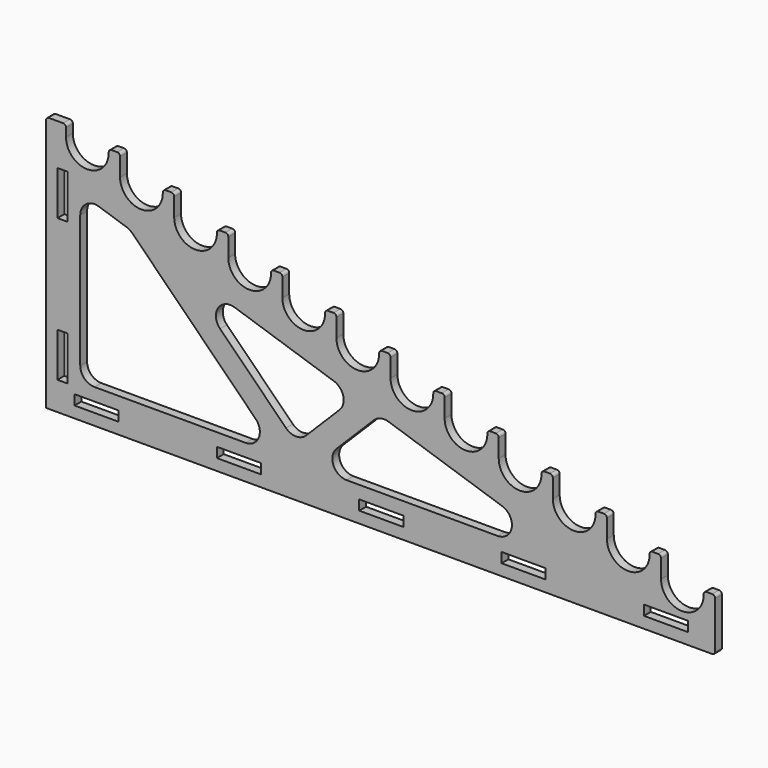
from build123d import *

# Parameters (mm, degrees)
F1_DEPTH = 3
F2_R     = 1
F3_W     = 15.5
F3_H     = 3.5
F3_W_2   = 3.5
F3_H_2   = 15.5
F4_DEPTH = 25


with BuildPart() as f1:
    # F0 (on Front) → F1 (new body)
    with BuildSketch(Plane.XZ):
        with BuildLine():
            Line((0, 90), (0, 0))
            Line((0, 0), (235, 0))
            Line((235, 0), (235, 17.5337082297))
            ThreePointArc((235, 17.5337082297), (234.7071067812, 18.2408150109), (234, 18.5337082297))
            Line((234, 18.5337082297), (232, 18.5337082297))
            ThreePointArc((232, 18.5337082297), (231.2928932188, 18.2408150109), (231, 17.5337082297))
            Line((231, 17.5337082297), (231, 17.3050220176))
            ThreePointArc((231, 17.3050220176), (223.5, 9.8050220176), (216, 17.3050220176))
            Line((216, 17.3050220176), (216, 21.3050220176))
            Line((216, 21.3050220176), (216, 23.7787062281))
            ThreePointArc((216, 23.7787062281), (215.7071067812, 24.4858130093), (215, 24.7787062281))
            Line((215, 24.7787062281), (213, 24.7787062281))
            ThreePointArc((213, 24.7787062281), (212.2928932188, 24.4858130093), (212, 23.7787062281))
            Line((212, 23.7787062281), (212, 23.550020016))
            ThreePointArc((212, 23.550020016), (204.5, 16.050020016), (197, 23.550020016))
            Line((197, 23.550020016), (197, 27.550020016))
            Line((197, 27.550020016), (197, 30.0237042265))
            ThreePointArc((197, 30.0237042265), (196.7071067812, 30.7308110077), (196, 31.0237042265))
            Line((196, 31.0237042265), (194, 31.0237042265))
            ThreePointArc((194, 31.0237042265), (193.2928932188, 30.7308110077), (193, 30.0237042265))
            Line((193, 30.0237042265), (193, 29.7950180144))
            ThreePointArc((193, 29.7950180144), (185.5, 22.2950180144), (178, 29.7950180144))
            Line((178, 29.7950180144), (178, 33.7950180144))
            Line((178, 33.7950180144), (178, 36.2687022249))
            ThreePointArc((178, 36.2687022249), (177.7071067812, 36.9758090061), (177, 37.2687022249))
            Line((177, 37.2687022249), (175, 37.2687022249))
            ThreePointArc((175, 37.2687022249), (174.2928932188, 36.9758090061), (174, 36.2687022249))
            Line((174, 36.2687022249), (174, 36.0400160128))
            ThreePointArc((174, 36.0400160128), (166.5, 28.5400160128), (159, 36.0400160128))
            Line((159, 36.0400160128), (159, 40.0400160128))
            Line((159, 40.0400160128), (159, 42.5137002233))
            ThreePointArc((159, 42.5137002233), (158.7071067812, 43.2208070045), (158, 43.5137002233))
            Line((158, 43.5137002233), (156, 43.5137002233))
            ThreePointArc((156, 43.5137002233), (155.2928932188, 43.2208070045), (155, 42.5137002233))
            Line((155, 42.5137002233), (155, 42.2850140112))
            ThreePointArc((155, 42.2850140112), (147.5, 34.7850140112), (140, 42.2850140112))
            Line((140, 42.2850140112), (140, 46.2850140112))
            Line((140, 46.2850140112), (140, 48.7586982217))
            ThreePointArc((140, 48.7586982217), (139.7071067812, 49.4658050029), (139, 49.7586982217))
            Line((139, 49.7586982217), (137, 49.7586982217))
            ThreePointArc((137, 49.7586982217), (136.2928932188, 49.4658050029), (136, 48.7586982217))
            Line((136, 48.7586982217), (136, 48.5300120096))
            ThreePointArc((136, 48.5300120096), (128.5, 41.0300120096), (121, 48.5300120096))
            Line((121, 48.5300120096), (121, 52.5300120096))
            Line((121, 52.5300120096), (121, 55.0036962201))
            ThreePointArc((121, 55.0036962201), (120.7071067812, 55.7108030013), (120, 56.0036962201))
            Line((120, 56.0036962201), (118, 56.0036962201))
            ThreePointArc((118, 56.0036962201), (117.2928932188, 55.7108030013), (117, 55.0036962201))
            Line((117, 55.0036962201), (117, 54.775010008))
            ThreePointArc((117, 54.775010008), (109.5, 47.275010008), (102, 54.775010008))
            Line((102, 54.775010008), (102, 58.775010008))
            Line((102, 58.775010008), (102, 61.2451730918))
            ThreePointArc((102, 61.2451730918), (101.7058629727, 61.9535214974), (100.9964850724, 62.2451669144))
            Line((100.9964850724, 62.2451669144), (98.9964850724, 62.2381370157))
            ThreePointArc((98.9964850724, 62.2381370157), (98.2916515943, 61.9440061658), (98, 61.2381431931))
            Line((98, 61.2381431931), (98, 61.0200080064))
            ThreePointArc((98, 61.0200080064), (90.5, 53.5200080064), (83, 61.0200080064))
            Line((83, 61.0200080064), (83, 65.0200080064))
            Line((83, 65.0200080064), (83, 67.4936922169))
            ThreePointArc((83, 67.4936922169), (82.7071067812, 68.2007989981), (82, 68.4936922169))
            Line((82, 68.4936922169), (80, 68.4936922169))
            ThreePointArc((80, 68.4936922169), (79.2928932188, 68.2007989981), (79, 67.4936922169))
            Line((79, 67.4936922169), (79, 67.2650060048))
            ThreePointArc((79, 67.2650060048), (71.5, 59.7650060048), (64, 67.2650060048))
            Line((64, 67.2650060048), (64, 71.2650060048))
            Line((64, 71.2650060048), (64, 73.7351690886))
            ThreePointArc((64, 73.7351690886), (63.7058629727, 74.4435174942), (62.9964850724, 74.7351629112))
            Line((62.9964850724, 74.7351629112), (60.9964850724, 74.7281330125))
            ThreePointArc((60.9964850724, 74.7281330125), (60.2916515943, 74.4340021625), (60, 73.7281391899))
            Line((60, 73.7281391899), (60, 73.5100040032))
            ThreePointArc((60, 73.5100040032), (52.5, 66.0100040032), (45, 73.5100040032))
            Line((45, 73.5100040032), (45, 77.5100040032))
            Line((45, 77.5100040032), (45, 79.980167087))
            ThreePointArc((45, 79.980167087), (44.7058629727, 80.6885154926), (43.9964850724, 80.9801609096))
            Line((43.9964850724, 80.9801609096), (41.9964850724, 80.9731310109))
            ThreePointArc((41.9964850724, 80.9731310109), (41.2916515943, 80.6790001609), (41, 79.9731371883))
            Line((41, 79.9731371883), (41, 79.7550020016))
            ThreePointArc((41, 79.7550020016), (33.5, 72.2550020016), (26, 79.7550020016))
            Line((26, 79.7550020016), (26, 83.7550020016))
            Line((26, 83.7550020016), (26, 86.2251650854))
            ThreePointArc((26, 86.2251650854), (25.7058629727, 86.933513491), (24.9964850724, 87.225158908))
            Line((24.9964850724, 87.225158908), (22.9964850724, 87.2181290093))
            ThreePointArc((22.9964850724, 87.2181290093), (22.2916515943, 86.9239981593), (22, 86.2181351867))
            Line((22, 86.2181351867), (22, 86))
            ThreePointArc((22, 86), (14.5, 78.5), (7, 86))
            Line((7, 86), (7, 89))
            ThreePointArc((7, 89), (6.7071067812, 89.7071067812), (6, 90))
            Line((6, 90), (0, 90))
        make_face()
        with BuildLine():
            ThreePointArc((17, 12), (13.4644660941, 13.4644660941), (12, 17))
            Line((12, 17), (12, 63.5552642114))
            ThreePointArc((12, 63.5552642114), (14.0679569834, 67.6053412167), (18.5612494996, 68.3052642114))
            Line((18.5612494996, 68.3052642114), (28.2995777656, 65.1044304993))
            ThreePointArc((28.2995777656, 65.1044304993), (29.3580672309, 64.6131824005), (30.273862172, 63.8899644052))
            Line((30.273862172, 63.8899644052), (73.6282926713, 20.5355339059))
            ThreePointArc((73.6282926713, 20.5355339059), (74.7121564279, 15.0865828382), (70.0927587654, 12))
            Line((70.0927587654, 12), (17, 12))
        make_face(mode=Mode.SUBTRACT)
        with BuildLine():
            Line((103.0593050185, 32.8954784413), (91.3562147326, 21.1923881554))
            ThreePointArc((91.3562147326, 21.1923881554), (87.8206808267, 19.7279220614), (84.2851469208, 21.1923881554))
            Line((84.2851469208, 21.1923881554), (61.1221171694, 44.3554179068))
            ThreePointArc((61.1221171694, 44.3554179068), (60.3988991741, 50.5106907776), (66.2189005749, 52.6409518128))
            Line((66.2189005749, 52.6409518128), (101.0850206122, 41.1810123472))
            ThreePointArc((101.0850206122, 41.1810123472), (104.3875986483, 37.589969509), (103.0593050185, 32.8954784413))
        make_face(mode=Mode.SUBTRACT)
        with BuildLine():
            ThreePointArc((160.202611153, 21.75), (163.578466068, 16.209430585), (158.6413616534, 12))
            Line((158.6413616534, 12), (105.5486028881, 12))
            ThreePointArc((105.5486028881, 12), (100.9292052255, 15.0865828382), (102.0130689821, 20.5355339059))
            Line((102.0130689821, 20.5355339059), (115.1469251322, 33.669390056))
            ThreePointArc((115.1469251322, 33.669390056), (117.5235018764, 34.9976836858), (120.2437085377, 34.88385615))
            Line((120.2437085377, 34.88385615), (160.202611153, 21.75))
        make_face(mode=Mode.SUBTRACT)
    extrude(amount=F1_DEPTH)

    # F2
    f2_edges = [f1.edges().sort_by_distance(p)[0] for p in [
        (235, -1.5, 0),
        (0, -1.5, 90),
    ]]
    fillet(f2_edges, radius=F2_R)

    # F3 (on face) → F4 (cut)
    with BuildSketch(Plane.XZ.offset(3)):
        with Locations((17.75, 5.75)):
            Rectangle(F3_W, F3_H)
        with Locations((5.75, 17.75)):
            Rectangle(F3_W_2, F3_H_2)
        with Locations((5.75, 67.75)):
            Rectangle(F3_W_2, F3_H_2)
        with Locations((67.75, 5.75)):
            Rectangle(F3_W, F3_H)
        with Locations((117.75, 5.75)):
            Rectangle(F3_W, F3_H)
        with Locations((167.75, 5.75)):
            Rectangle(F3_W, F3_H)
        with Locations((217.75, 5.75)):
            Rectangle(F3_W, F3_H)
    extrude(amount=-F4_DEPTH, mode=Mode.SUBTRACT)


solid = f1.part
